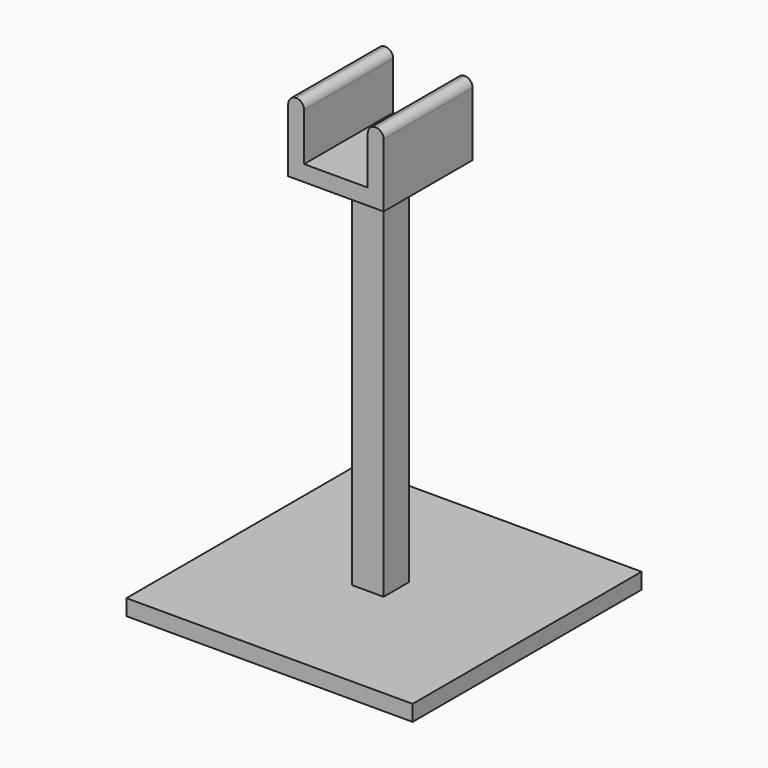
from build123d import *

# Parameters (mm, degrees)
F0_W     = 914.4
F0_H     = 914.4
F1_DEPTH = 50.8
F2_W     = 101.6
F2_H     = 101.6
F3_DEPTH = 1219.2
F4_W     = 304.8
F4_H     = 355.6
F5_DEPTH = 228.6
F6_W     = 203.2
F6_H     = 355.6
F7_DEPTH = 177.8
F8_R     = 25.39999


# Not quite as in the source:
# - a fillet or chamfer is up to 0.001 mm smaller than in the source, because OpenCascade refuses the exact size
# - a feature names something its author has since deleted; it is built from what else it names


with BuildPart() as f1:
    # F0 (on Top) → F1 (new body)
    with BuildSketch(Plane.XY):
        with Locations((11.3640455229, 0)):
            Rectangle(F0_W, F0_H)
    extrude(amount=F1_DEPTH)

    # F2 (on face) → F3 (join)
    with BuildSketch(Plane(origin=(0, 0, 0), x_dir=(1, 0, 0), z_dir=(0, 0, -1))):
        Rectangle(F2_W, F2_H)
    extrude(amount=-F3_DEPTH)

    # F4 (on face) → F5 (join)
    with BuildSketch(Plane.XY.offset(1219.2)):
        Rectangle(F4_W, F4_H)
    extrude(amount=F5_DEPTH)

    # F6 (on face) → F7 (cut)
    with BuildSketch(Plane.XY.offset(1447.8)):
        Rectangle(F6_W, F6_H)
    extrude(amount=-F7_DEPTH, mode=Mode.SUBTRACT)

    # F8 (radius 25.4 in the source; OpenCascade refuses exactly that, so slightly less here)
    f8_edges = [f1.edges().sort_by_distance(p)[0] for p in [
        (-152.4, 0, 1447.8),
        (-101.6, 0, 1447.8),
        (101.6, 0, 1447.8),
        (152.4, 0, 1447.8),
    ]]
    fillet(f8_edges, radius=F8_R)


solid = f1.part
